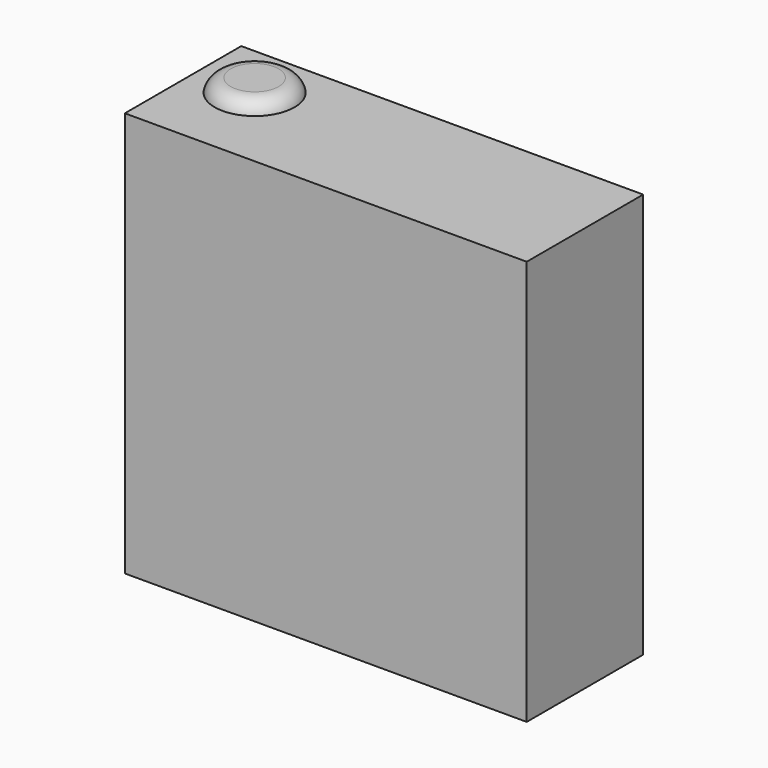
from build123d import *

# Parameters (mm, degrees)
F0_W     = 125.5502849817
F0_H     = 126.5566982329
F1_DEPTH = 45.466
F2_R     = 12.4740683963
F3_DEPTH = 4.064


# Not quite as in the source:
# - a fillet or chamfer that OpenCascade refuses, or shapes differently, is made with other operations: its cross-section is extruded or revolved along the edge and cut away or added


with BuildPart() as f1:
    # F0 (on Front) → F1 (new body)
    with BuildSketch(Plane.XZ):
        with Locations((3.0192434788, -2.1386351436)):
            Rectangle(F0_W, F0_H)
    extrude(amount=F1_DEPTH)

    # F2 (on face) → F3 (join)
    with BuildSketch(Plane.XY.offset(61.1397139728)):
        with Locations((-41.892029345, -17.1090569347)):
            Circle(F2_R)
    extrude(amount=F3_DEPTH)

    # F4: fillet of radius 5.08 on 1 edges, made by hand

    # F4_s1 → F4_t2 (revolve, cut)
    with BuildSketch(Plane.XZ.offset(17.1090569347)):
        with BuildLine():
            ThreePointArc((-29.4179609488, 61.1397139728), (-31.1824500034, 64.0586650526), (-34.3953241061, 65.2037139728))
            Line((-34.3953241061, 65.2037139728), (-29.4179609488, 65.2037139728))
            Line((-29.4179609488, 65.2037139728), (-29.4179609488, 61.1397139728))
        make_face()
    revolve(axis=Axis((-41.892029345, -17.1090569347, 65.2037139728), (0, 0, 1)), mode=Mode.SUBTRACT)


solid = f1.part
